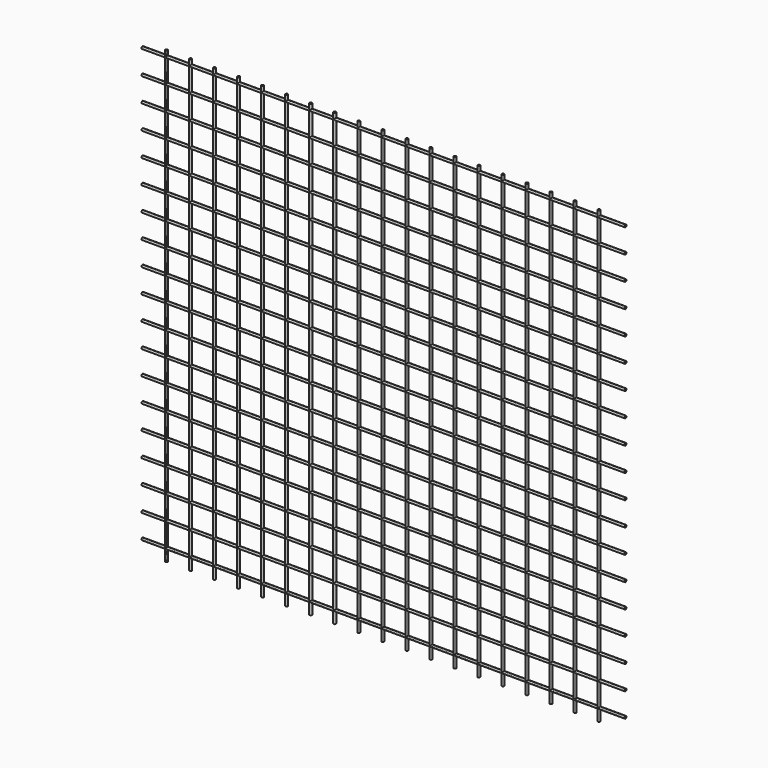
from build123d import *

# Parameters (mm, degrees)
F3_DEPTH = 1004.9
F4_DEPTH = 936.8


# Not quite as in the source:
# - a feature names something its author has since deleted; it is built from what else it names


with BuildPart() as f3:
    # F0 (on Right) → F3 (new body)
    with BuildSketch(Plane.YZ):
        with BuildLine():
            Line((-8.4, 416.895691), (-8.4, 421.895691))
            ThreePointArc((-8.4, 421.895691), (-10.9, 419.395691), (-8.4, 416.895691))
        make_face()
        with BuildLine():
            ThreePointArc((-5.9, 419.395691), (-6.632233, 421.163458), (-8.4, 421.895691))
            Line((-8.4, 421.895691), (-8.4, 416.895691))
            ThreePointArc((-8.4, 416.895691), (-6.632233, 417.627924), (-5.9, 419.395691))
        make_face()
    extrude(amount=F3_DEPTH)



with BuildPart() as f3b:
    # F0 (on Right) → F3, piece 2 (new body)
    with BuildSketch(Plane.YZ):
        with BuildLine():
            ThreePointArc((-5.9, 369.395691), (-6.632233, 371.163458), (-8.4, 371.895691))
            Line((-8.4, 371.895691), (-8.4, 366.895691))
            ThreePointArc((-8.4, 366.895691), (-6.632233, 367.627924), (-5.9, 369.395691))
        make_face()
        with BuildLine():
            Line((-8.4, 366.895691), (-8.4, 371.895691))
            ThreePointArc((-8.4, 371.895691), (-10.9, 369.395691), (-8.4, 366.895691))
        make_face()
    extrude(amount=F3_DEPTH)


with BuildPart() as f3c:
    # F0 (on Right) → F3, piece 3 (new body)
    with BuildSketch(Plane.YZ):
        with BuildLine():
            ThreePointArc((-5.9, 319.395691), (-6.632233, 321.163458), (-8.4, 321.895691))
            Line((-8.4, 321.895691), (-8.4, 316.895691))
            ThreePointArc((-8.4, 316.895691), (-6.632233, 317.627924), (-5.9, 319.395691))
        make_face()
        with BuildLine():
            Line((-8.4, 316.895691), (-8.4, 321.895691))
            ThreePointArc((-8.4, 321.895691), (-10.9, 319.395691), (-8.4, 316.895691))
        make_face()
    extrude(amount=F3_DEPTH)


with BuildPart() as f3d:
    # F0 (on Right) → F3, piece 4 (new body)
    with BuildSketch(Plane.YZ):
        with BuildLine():
            ThreePointArc((-5.9, 269.395691), (-6.632233, 271.163458), (-8.4, 271.895691))
            Line((-8.4, 271.895691), (-8.4, 266.895691))
            ThreePointArc((-8.4, 266.895691), (-6.632233, 267.627924), (-5.9, 269.395691))
        make_face()
        with BuildLine():
            Line((-8.4, 266.895691), (-8.4, 271.895691))
            ThreePointArc((-8.4, 271.895691), (-10.9, 269.395691), (-8.4, 266.895691))
        make_face()
    extrude(amount=F3_DEPTH)


with BuildPart() as f3e:
    # F0 (on Right) → F3, piece 5 (new body)
    with BuildSketch(Plane.YZ):
        with BuildLine():
            Line((-8.4, 216.895691), (-8.4, 221.895691))
            ThreePointArc((-8.4, 221.895691), (-10.9, 219.395691), (-8.4, 216.895691))
        make_face()
        with BuildLine():
            ThreePointArc((-5.9, 219.395691), (-6.632233, 221.163458), (-8.4, 221.895691))
            Line((-8.4, 221.895691), (-8.4, 216.895691))
            ThreePointArc((-8.4, 216.895691), (-6.632233, 217.627924), (-5.9, 219.395691))
        make_face()
    extrude(amount=F3_DEPTH)


with BuildPart() as f3f:
    # F0 (on Right) → F3, piece 6 (new body)
    with BuildSketch(Plane.YZ):
        with BuildLine():
            ThreePointArc((-5.9, 169.395691), (-6.632233, 171.163458), (-8.4, 171.895691))
            Line((-8.4, 171.895691), (-8.4, 166.895691))
            ThreePointArc((-8.4, 166.895691), (-6.632233, 167.627924), (-5.9, 169.395691))
        make_face()
        with BuildLine():
            Line((-8.4, 166.895691), (-8.4, 171.895691))
            ThreePointArc((-8.4, 171.895691), (-10.9, 169.395691), (-8.4, 166.895691))
        make_face()
    extrude(amount=F3_DEPTH)


with BuildPart() as f3g:
    # F0 (on Right) → F3, piece 7 (new body)
    with BuildSketch(Plane.YZ):
        with BuildLine():
            ThreePointArc((-5.9, -30.604309), (-6.632233, -28.836542), (-8.4, -28.104309))
            Line((-8.4, -28.104309), (-8.4, -33.104309))
            ThreePointArc((-8.4, -33.104309), (-6.632233, -32.372076), (-5.9, -30.604309))
        make_face()
        with BuildLine():
            Line((-8.4, -33.104309), (-8.4, -28.104309))
            ThreePointArc((-8.4, -28.104309), (-10.9, -30.604309), (-8.4, -33.104309))
        make_face()
    extrude(amount=F3_DEPTH)


with BuildPart() as f3h:
    # F0 (on Right) → F3, piece 8 (new body)
    with BuildSketch(Plane.YZ):
        with BuildLine():
            Line((-8.4, 16.895691), (-8.4, 21.895691))
            ThreePointArc((-8.4, 21.895691), (-10.9, 19.395691), (-8.4, 16.895691))
        make_face()
        with BuildLine():
            ThreePointArc((-5.9, 19.395691), (-6.632233, 21.163458), (-8.4, 21.895691))
            Line((-8.4, 21.895691), (-8.4, 16.895691))
            ThreePointArc((-8.4, 16.895691), (-6.632233, 17.627924), (-5.9, 19.395691))
        make_face()
    extrude(amount=F3_DEPTH)


with BuildPart() as f3i:
    # F0 (on Right) → F3, piece 9 (new body)
    with BuildSketch(Plane.YZ):
        with BuildLine():
            ThreePointArc((-5.9, 119.395691), (-6.632233, 121.163458), (-8.4, 121.895691))
            Line((-8.4, 121.895691), (-8.4, 116.895691))
            ThreePointArc((-8.4, 116.895691), (-6.632233, 117.627924), (-5.9, 119.395691))
        make_face()
        with BuildLine():
            Line((-8.4, 116.895691), (-8.4, 121.895691))
            ThreePointArc((-8.4, 121.895691), (-10.9, 119.395691), (-8.4, 116.895691))
        make_face()
    extrude(amount=F3_DEPTH)


with BuildPart() as f3j:
    # F0 (on Right) → F3, piece 10 (new body)
    with BuildSketch(Plane.YZ):
        with BuildLine():
            ThreePointArc((-8.4, -178.104309), (-10.9, -180.604309), (-8.4, -183.104309))
            Line((-8.4, -183.104309), (-8.4, -178.104309))
        make_face()
        with BuildLine():
            Line((-8.4, -178.104309), (-8.4, -183.104309))
            ThreePointArc((-8.4, -183.104309), (-6.632233, -182.372076), (-5.9, -180.604309))
            ThreePointArc((-5.9, -180.604309), (-6.632233, -178.836542), (-8.4, -178.104309))
        make_face()
    extrude(amount=F3_DEPTH)


with BuildPart() as f3k:
    # F0 (on Right) → F3, piece 11 (new body)
    with BuildSketch(Plane.YZ):
        with BuildLine():
            ThreePointArc((-5.9, 69.395691), (-6.632233, 71.163458), (-8.4, 71.895691))
            Line((-8.4, 71.895691), (-8.4, 66.895691))
            ThreePointArc((-8.4, 66.895691), (-6.632233, 67.627924), (-5.9, 69.395691))
        make_face()
        with BuildLine():
            Line((-8.4, 66.895691), (-8.4, 71.895691))
            ThreePointArc((-8.4, 71.895691), (-10.9, 69.395691), (-8.4, 66.895691))
        make_face()
    extrude(amount=F3_DEPTH)


with BuildPart() as f3l:
    # F0 (on Right) → F3, piece 12 (new body)
    with BuildSketch(Plane.YZ):
        with BuildLine():
            ThreePointArc((-8.4, -128.104309), (-10.9, -130.604309), (-8.4, -133.104309))
            Line((-8.4, -133.104309), (-8.4, -128.104309))
        make_face()
        with BuildLine():
            Line((-8.4, -128.104309), (-8.4, -133.104309))
            ThreePointArc((-8.4, -133.104309), (-6.632233, -132.372076), (-5.9, -130.604309))
            ThreePointArc((-5.9, -130.604309), (-6.632233, -128.836542), (-8.4, -128.104309))
        make_face()
    extrude(amount=F3_DEPTH)


with BuildPart() as f3m:
    # F0 (on Right) → F3, piece 13 (new body)
    with BuildSketch(Plane.YZ):
        with BuildLine():
            ThreePointArc((-8.4, -78.104309), (-10.9, -80.604309), (-8.4, -83.104309))
            Line((-8.4, -83.104309), (-8.4, -78.104309))
        make_face()
        with BuildLine():
            Line((-8.4, -78.104309), (-8.4, -83.104309))
            ThreePointArc((-8.4, -83.104309), (-6.632233, -82.372076), (-5.9, -80.604309))
            ThreePointArc((-5.9, -80.604309), (-6.632233, -78.836542), (-8.4, -78.104309))
        make_face()
    extrude(amount=F3_DEPTH)


with BuildPart() as f3n:
    # F0 (on Right) → F3, piece 14 (new body)
    with BuildSketch(Plane.YZ):
        with BuildLine():
            ThreePointArc((-8.4, -328.104309), (-10.9, -330.604309), (-8.4, -333.104309))
            Line((-8.4, -333.104309), (-8.4, -328.104309))
        make_face()
        with BuildLine():
            Line((-8.4, -328.104309), (-8.4, -333.104309))
            ThreePointArc((-8.4, -333.104309), (-6.632233, -332.372076), (-5.9, -330.604309))
            ThreePointArc((-5.9, -330.604309), (-6.632233, -328.836542), (-8.4, -328.104309))
        make_face()
    extrude(amount=F3_DEPTH)


with BuildPart() as f3o:
    # F0 (on Right) → F3, piece 15 (new body)
    with BuildSketch(Plane.YZ):
        with BuildLine():
            ThreePointArc((-8.4, -278.104309), (-10.9, -280.604309), (-8.4, -283.104309))
            Line((-8.4, -283.104309), (-8.4, -278.104309))
        make_face()
        with BuildLine():
            Line((-8.4, -278.104309), (-8.4, -283.104309))
            ThreePointArc((-8.4, -283.104309), (-6.632233, -282.372076), (-5.9, -280.604309))
            ThreePointArc((-5.9, -280.604309), (-6.632233, -278.836542), (-8.4, -278.104309))
        make_face()
    extrude(amount=F3_DEPTH)


with BuildPart() as f3p:
    # F0 (on Right) → F3, piece 16 (new body)
    with BuildSketch(Plane.YZ):
        with BuildLine():
            ThreePointArc((-8.4, -228.104309), (-10.9, -230.604309), (-8.4, -233.104309))
            Line((-8.4, -233.104309), (-8.4, -228.104309))
        make_face()
        with BuildLine():
            Line((-8.4, -228.104309), (-8.4, -233.104309))
            ThreePointArc((-8.4, -233.104309), (-6.632233, -232.372076), (-5.9, -230.604309))
            ThreePointArc((-5.9, -230.604309), (-6.632233, -228.836542), (-8.4, -228.104309))
        make_face()
    extrude(amount=F3_DEPTH)


with BuildPart() as f3q:
    # F0 (on Right) → F3, piece 17 (new body)
    with BuildSketch(Plane.YZ):
        with BuildLine():
            Line((-8.4, -378.104309), (-8.4, -383.104309))
            ThreePointArc((-8.4, -383.104309), (-6.632233, -382.372076), (-5.9, -380.604309))
            ThreePointArc((-5.9, -380.604309), (-6.632233, -378.836542), (-8.4, -378.104309))
        make_face()
        with BuildLine():
            ThreePointArc((-8.4, -378.104309), (-10.9, -380.604309), (-8.4, -383.104309))
            Line((-8.4, -383.104309), (-8.4, -378.104309))
        make_face()
    extrude(amount=F3_DEPTH)


with BuildPart() as f3r:
    # F0 (on Right) → F3, piece 18 (new body)
    with BuildSketch(Plane.YZ):
        with BuildLine():
            Line((-8.4, -428.104309), (-8.4, -433.104309))
            ThreePointArc((-8.4, -433.104309), (-6.632233, -432.372076), (-5.9, -430.604309))
            ThreePointArc((-5.9, -430.604309), (-6.632233, -428.836542), (-8.4, -428.104309))
        make_face()
        with BuildLine():
            ThreePointArc((-8.4, -428.104309), (-10.9, -430.604309), (-8.4, -433.104309))
            Line((-8.4, -433.104309), (-8.4, -428.104309))
        make_face()
    extrude(amount=F3_DEPTH)


with BuildPart() as f3s:
    # F0 (on Right) → F3, piece 19 (new body)
    with BuildSketch(Plane.YZ):
        with BuildLine():
            ThreePointArc((-8.4, -478.104309), (-10.167767, -478.836542), (-10.9, -480.604309))
            Line((-10.9, -480.604309), (-8.4, -480.604309))
            Line((-8.4, -480.604309), (-8.4, -478.104309))
        make_face()
        with BuildLine():
            Line((-8.4, -480.604309), (-5.9, -480.604309))
            ThreePointArc((-5.9, -480.604309), (-6.632233, -478.836542), (-8.4, -478.104309))
            Line((-8.4, -478.104309), (-8.4, -480.604309))
        make_face()
        with BuildLine():
            Line((-8.4, -480.604309), (-10.9, -480.604309))
            ThreePointArc((-10.9, -480.604309), (-10.167767, -482.372076), (-8.4, -483.104309))
            Line((-8.4, -483.104309), (-8.4, -480.604309))
        make_face()
        with BuildLine():
            ThreePointArc((-8.4, -483.104309), (-6.632233, -482.372076), (-5.9, -480.604309))
            Line((-5.9, -480.604309), (-8.4, -480.604309))
            Line((-8.4, -480.604309), (-8.4, -483.104309))
        make_face()
    extrude(amount=F3_DEPTH)


with BuildPart() as f3_1:
    add(f3.part)

    add(f3b.part)  # F4 merges F3b

    add(f3c.part)  # F4 merges F3c

    add(f3d.part)  # F4 merges F3d

    add(f3e.part)  # F4 merges F3e

    add(f3f.part)  # F4 merges F3f

    add(f3g.part)  # F4 merges F3g

    add(f3h.part)  # F4 merges F3h

    add(f3i.part)  # F4 merges F3i

    add(f3j.part)  # F4 merges F3j

    add(f3k.part)  # F4 merges F3k

    add(f3l.part)  # F4 merges F3l

    add(f3m.part)  # F4 merges F3m

    add(f3n.part)  # F4 merges F3n

    add(f3o.part)  # F4 merges F3o

    add(f3p.part)  # F4 merges F3p

    add(f3q.part)  # F4 merges F3q

    add(f3r.part)  # F4 merges F3r

    add(f3s.part)  # F4 merges F3s
    # F2 (on offset) → F4 (join)
    with BuildSketch(Plane.XY.offset(431.19)):
        with BuildLine():
            Line((50, -8.4), (50, -10.9))
            ThreePointArc((50, -10.9), (51.767767, -10.167767), (52.5, -8.4))
            Line((52.5, -8.4), (50, -8.4))
        make_face()
        with BuildLine():
            ThreePointArc((47.5, -8.4), (48.232233, -10.167767), (50, -10.9))
            Line((50, -10.9), (50, -8.4))
            Line((50, -8.4), (47.5, -8.4))
        make_face()
        with BuildLine():
            Line((47.5, -8.4), (50, -8.4))
            Line((50, -8.4), (50, -5.9))
            ThreePointArc((50, -5.9), (48.232233, -6.632233), (47.5, -8.4))
        make_face()
        with BuildLine():
            Line((50, -5.9), (50, -8.4))
            Line((50, -8.4), (52.5, -8.4))
            ThreePointArc((52.5, -8.4), (51.767767, -6.632233), (50, -5.9))
        make_face()
        with BuildLine():
            ThreePointArc((202.5, -8.4), (200, -5.9), (197.5, -8.4))
            Line((197.5, -8.4), (202.5, -8.4))
        make_face()
        with BuildLine():
            ThreePointArc((152.5, -8.4), (150, -5.9), (147.5, -8.4))
            Line((147.5, -8.4), (152.5, -8.4))
        make_face()
        with BuildLine():
            Line((202.5, -8.4), (197.5, -8.4))
            ThreePointArc((197.5, -8.4), (200, -10.9), (202.5, -8.4))
        make_face()
        with BuildLine():
            Line((152.5, -8.4), (147.5, -8.4))
            ThreePointArc((147.5, -8.4), (150, -10.9), (152.5, -8.4))
        make_face()
        with BuildLine():
            Line((102.5, -8.4), (97.5, -8.4))
            ThreePointArc((97.5, -8.4), (100, -10.9), (102.5, -8.4))
        make_face()
        with BuildLine():
            ThreePointArc((102.5, -8.4), (100, -5.9), (97.5, -8.4))
            Line((97.5, -8.4), (102.5, -8.4))
        make_face()
        with BuildLine():
            Line((352.5, -8.4), (347.5, -8.4))
            ThreePointArc((347.5, -8.4), (350, -10.9), (352.5, -8.4))
        make_face()
        with BuildLine():
            Line((252.5, -8.4), (247.5, -8.4))
            ThreePointArc((247.5, -8.4), (250, -10.9), (252.5, -8.4))
        make_face()
        with BuildLine():
            Line((302.5, -8.4), (297.5, -8.4))
            ThreePointArc((297.5, -8.4), (300, -10.9), (302.5, -8.4))
        make_face()
        with BuildLine():
            Line((502.5, -8.4), (497.5, -8.4))
            ThreePointArc((497.5, -8.4), (500, -10.9), (502.5, -8.4))
        make_face()
        with BuildLine():
            ThreePointArc((452.5, -8.4), (450, -5.9), (447.5, -8.4))
            Line((447.5, -8.4), (452.5, -8.4))
        make_face()
        with BuildLine():
            ThreePointArc((647.5, -8.4), (650, -10.9), (652.5, -8.4))
            Line((652.5, -8.4), (647.5, -8.4))
        make_face()
        with BuildLine():
            ThreePointArc((252.5, -8.4), (250, -5.9), (247.5, -8.4))
            Line((247.5, -8.4), (252.5, -8.4))
        make_face()
        with BuildLine():
            ThreePointArc((502.5, -8.4), (500, -5.9), (497.5, -8.4))
            Line((497.5, -8.4), (502.5, -8.4))
        make_face()
        with BuildLine():
            ThreePointArc((597.5, -8.4), (600, -10.9), (602.5, -8.4))
            Line((602.5, -8.4), (597.5, -8.4))
        make_face()
        with BuildLine():
            Line((402.5, -8.4), (397.5, -8.4))
            ThreePointArc((397.5, -8.4), (400, -10.9), (402.5, -8.4))
        make_face()
        with BuildLine():
            Line((547.5, -8.4), (552.5, -8.4))
            ThreePointArc((552.5, -8.4), (550, -5.9), (547.5, -8.4))
        make_face()
        with BuildLine():
            Line((647.5, -8.4), (652.5, -8.4))
            ThreePointArc((652.5, -8.4), (650, -5.9), (647.5, -8.4))
        make_face()
        with BuildLine():
            Line((452.5, -8.4), (447.5, -8.4))
            ThreePointArc((447.5, -8.4), (450, -10.9), (452.5, -8.4))
        make_face()
        with BuildLine():
            ThreePointArc((697.5, -8.4), (700, -10.9), (702.5, -8.4))
            Line((702.5, -8.4), (697.5, -8.4))
        make_face()
        with BuildLine():
            ThreePointArc((352.5, -8.4), (350, -5.9), (347.5, -8.4))
            Line((347.5, -8.4), (352.5, -8.4))
        make_face()
        with BuildLine():
            Line((697.5, -8.4), (702.5, -8.4))
            ThreePointArc((702.5, -8.4), (700, -5.9), (697.5, -8.4))
        make_face()
        with BuildLine():
            ThreePointArc((547.5, -8.4), (550, -10.9), (552.5, -8.4))
            Line((552.5, -8.4), (547.5, -8.4))
        make_face()
        with BuildLine():
            ThreePointArc((302.5, -8.4), (300, -5.9), (297.5, -8.4))
            Line((297.5, -8.4), (302.5, -8.4))
        make_face()
        with BuildLine():
            ThreePointArc((402.5, -8.4), (400, -5.9), (397.5, -8.4))
            Line((397.5, -8.4), (402.5, -8.4))
        make_face()
        with BuildLine():
            Line((597.5, -8.4), (602.5, -8.4))
            ThreePointArc((602.5, -8.4), (600, -5.9), (597.5, -8.4))
        make_face()
        with BuildLine():
            Line((847.5, -8.4), (852.5, -8.4))
            ThreePointArc((852.5, -8.4), (850, -5.9), (847.5, -8.4))
        make_face()
        with BuildLine():
            ThreePointArc((797.5, -8.4), (800, -10.9), (802.5, -8.4))
            Line((802.5, -8.4), (797.5, -8.4))
        make_face()
        with BuildLine():
            Line((947.5, -8.4), (952.5, -8.4))
            ThreePointArc((952.5, -8.4), (950, -5.9), (947.5, -8.4))
        make_face()
        with BuildLine():
            Line((897.5, -8.4), (902.5, -8.4))
            ThreePointArc((902.5, -8.4), (900, -5.9), (897.5, -8.4))
        make_face()
        with BuildLine():
            Line((797.5, -8.4), (802.5, -8.4))
            ThreePointArc((802.5, -8.4), (800, -5.9), (797.5, -8.4))
        make_face()
        with BuildLine():
            ThreePointArc((947.5, -8.4), (950, -10.9), (952.5, -8.4))
            Line((952.5, -8.4), (947.5, -8.4))
        make_face()
        with BuildLine():
            ThreePointArc((847.5, -8.4), (850, -10.9), (852.5, -8.4))
            Line((852.5, -8.4), (847.5, -8.4))
        make_face()
        with BuildLine():
            ThreePointArc((747.5, -8.4), (750, -10.9), (752.5, -8.4))
            Line((752.5, -8.4), (747.5, -8.4))
        make_face()
        with BuildLine():
            Line((747.5, -8.4), (752.5, -8.4))
            ThreePointArc((752.5, -8.4), (750, -5.9), (747.5, -8.4))
        make_face()
        with BuildLine():
            ThreePointArc((897.5, -8.4), (900, -10.9), (902.5, -8.4))
            Line((902.5, -8.4), (897.5, -8.4))
        make_face()
    extrude(amount=-F4_DEPTH)


solid = f3_1.part
